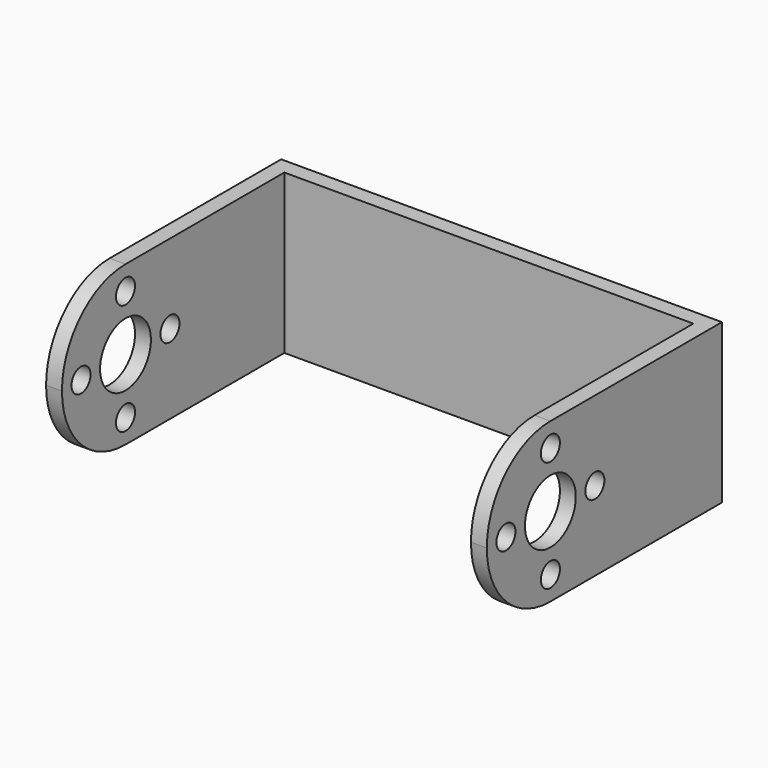
from build123d import *

# Parameters (mm, degrees)
F1_DEPTH = 20
F2_R     = 9.99999
F3_R     = 4
F3_R_2   = 1.5
F4_DEPTH = 55.501


# Not quite as in the source:
# - a fillet or chamfer is up to 0.001 mm smaller than in the source, because OpenCascade refuses the exact size


with BuildPart() as f1:
    # F0 (on Top) → F1 (new body)
    with BuildSketch(Plane.XY):
        Polygon((-27.75, 37), (-27.75, 0), (-25.75, 0), (-25.75, 35), (25.75, 35), (25.75, 0), (27.75, 0), (27.75, 37), align=None)
    extrude(amount=F1_DEPTH)

    # F2 (radius 10 in the source; OpenCascade refuses exactly that, so slightly less here)
    f2_edges = [f1.edges().sort_by_distance(p)[0] for p in [
        (-26.75, 0, 0),
        (-26.75, 0, 20),
        (26.75, 0, 0),
        (26.75, 0, 20),
    ]]
    fillet(f2_edges, radius=F2_R)

    # F3 (on face) → F4 (cut, through all)
    with BuildSketch(Plane(origin=(-27.75, 0, 0), x_dir=(0, -1, 0), z_dir=(-1, 0, 0))):
        with Locations((-10, 10)):
            Circle(F3_R)
        with Locations((-10, 3)):
            Circle(F3_R_2)
        with Locations((-10, 17)):
            Circle(F3_R_2)
        with Locations((-3, 10)):
            Circle(F3_R_2)
        with Locations((-17, 10)):
            Circle(F3_R_2)
    extrude(amount=-F4_DEPTH, mode=Mode.SUBTRACT)


solid = f1.part
